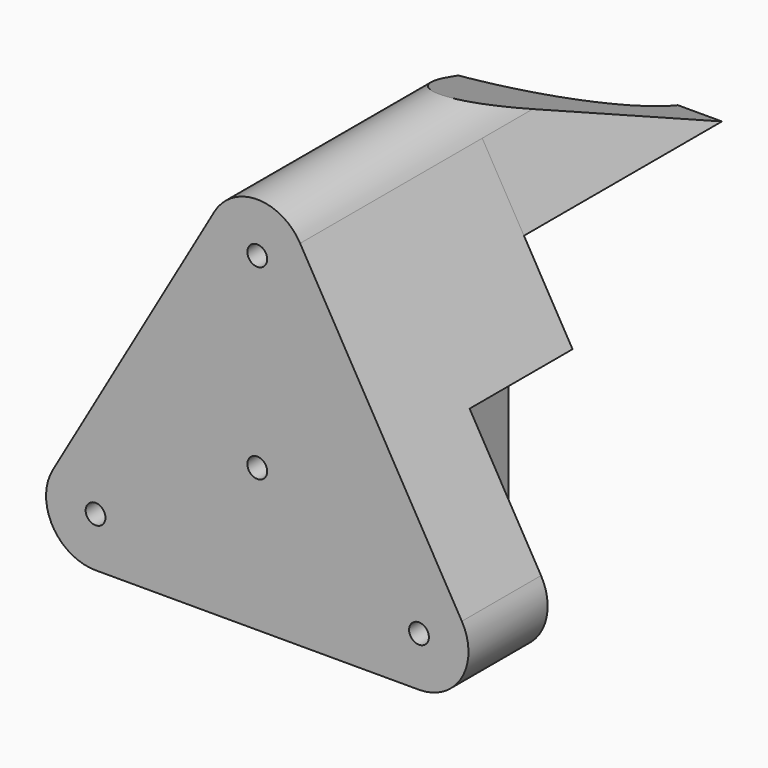
from build123d import *

# Parameters (mm, degrees)
F1_DEPTH  = 10
F3_D      = 2
F3_DEPTH  = 12
F3_TIP    = 0.600860619
F4_R      = 1
F5_DEPTH  = 13
F7_DEPTH  = 25
F9_DEPTH  = 9.8022701892
F11_DEPTH = 12.5


with BuildPart() as f1:
    # F0 (on Front) → F1 (new body)
    with BuildSketch(Plane.XZ):
        with BuildLine():
            Line((-4.3301270189, 21.3675134595), (-20.6698729811, -6.9337567297))
            ThreePointArc((-20.6698729811, -6.9337567297), (-20.6698729811, -11.9337567297), (-16.3397459622, -14.4337567297))
            Line((-16.3397459622, -14.4337567297), (16.3397459622, -14.4337567297))
            ThreePointArc((16.3397459622, -14.4337567297), (20.6698729811, -11.9337567297), (20.6698729811, -6.9337567297))
            Line((20.6698729811, -6.9337567297), (4.3301270189, 21.3675134595))
            ThreePointArc((4.3301270189, 21.3675134595), (0, 23.8675134595), (-4.3301270189, 21.3675134595))
        make_face()
    extrude(amount=F1_DEPTH)

    # F3
    with Locations(Plane.XZ.offset(10)):
        with Locations((0, 18.8675134595), (0, 0), (16.3397459622, -9.4337567297), (-16.3397459622, -9.4337567297)):
            Hole(F3_D / 2, depth=F3_DEPTH)
            with Locations((0, 0, -(F3_DEPTH + F3_TIP / 2))):  # 118° drill point
                Cone(0, F3_D / 2, F3_TIP, mode=Mode.SUBTRACT)

    # F4 (on face) → F5 (join)
    with BuildSketch(Plane(origin=(0, 0, 0), x_dir=(-1, 0, 0), z_dir=(0, 1, 0))):
        with BuildLine():
            Line((-7, 5.5662432703), (-7, -14.4337567297))
            Line((-7, -14.4337567297), (16.3397459622, -14.4337567297))
            ThreePointArc((16.3397459622, -14.4337567297), (20.6698729811, -11.9337567297), (20.6698729811, -6.9337567297))
            Line((20.6698729811, -6.9337567297), (4.3301270189, 21.3675134595))
            ThreePointArc((4.3301270189, 21.3675134595), (0, 23.8675134595), (-4.3301270189, 21.3675134595))
            Line((-4.3301270189, 21.3675134595), (-13.4529946162, 5.5662432703))
            Line((-13.4529946162, 5.5662432703), (-7, 5.5662432703))
        make_face()
        with Locations((16.3397459622, -9.4337567297)):
            Circle(F4_R, mode=Mode.SUBTRACT)
        Circle(F4_R, mode=Mode.SUBTRACT)
        with Locations((0, 18.8675134595)):
            Circle(F4_R, mode=Mode.SUBTRACT)
        with Locations((16.3397459622, -9.4337567297)):
            Circle(F4_R)
        Circle(F4_R)
        with Locations((0, 18.8675134595)):
            Circle(F4_R)
    extrude(amount=F5_DEPTH)

    # F6 (on face) → F7 (join)
    with BuildSketch(Plane(origin=(0, 13, 0), x_dir=(-1, 0, 0), z_dir=(0, 1, 0))):
        with BuildLine():
            Line((8.5455173281, 14.0662432703), (4.3301270189, 21.3675134595))
            ThreePointArc((4.3301270189, 21.3675134595), (0, 23.8675134595), (-4.3301270189, 21.3675134595))
            Line((-4.3301270189, 21.3675134595), (-8.5455173281, 14.0662432703))
            Line((-8.5455173281, 14.0662432703), (8.5455173281, 14.0662432703))
        make_face()
    extrude(amount=F7_DEPTH)

    # F8 (on face) → F9 (cut, through all)
    with BuildSketch(Plane(origin=(0, 0, 14.0662432703), x_dir=(1, 0, 0), z_dir=(0, 0, -1))):
        with BuildLine():
            Line((-8.5455173281, -38), (-8.5455173281, -20.0741813354))
            ThreePointArc((-8.5455173281, -20.0741813354), (-24.827324347, -44.9686543445), (4.0910069124, -38))
            Line((4.0910069124, -38), (-8.5455173281, -38))
        make_face()
        with BuildLine():
            ThreePointArc((4.0910069124, -38), (4.2102022324, -36.8778052582), (4.25, -35.75))
            ThreePointArc((4.25, -35.75), (0.6449933996, -25.6324835743), (-8.5455173281, -20.0741813354))
            Line((-8.5455173281, -20.0741813354), (-8.5455173281, -38))
            Line((-8.5455173281, -38), (4.0910069124, -38))
        make_face()
    extrude(amount=-F9_DEPTH, mode=Mode.SUBTRACT)

    # F10 (on Right) → F11 (cut, symmetric)
    with BuildSketch(Plane.YZ):
        Polygon((13, 23.8675134595), (38, 14.0662432703), (39, 14.0662432703), (39, 24.8675134595), (13, 24.8675134595), align=None)
    extrude(amount=F11_DEPTH, both=True, mode=Mode.SUBTRACT)


solid = f1.part
